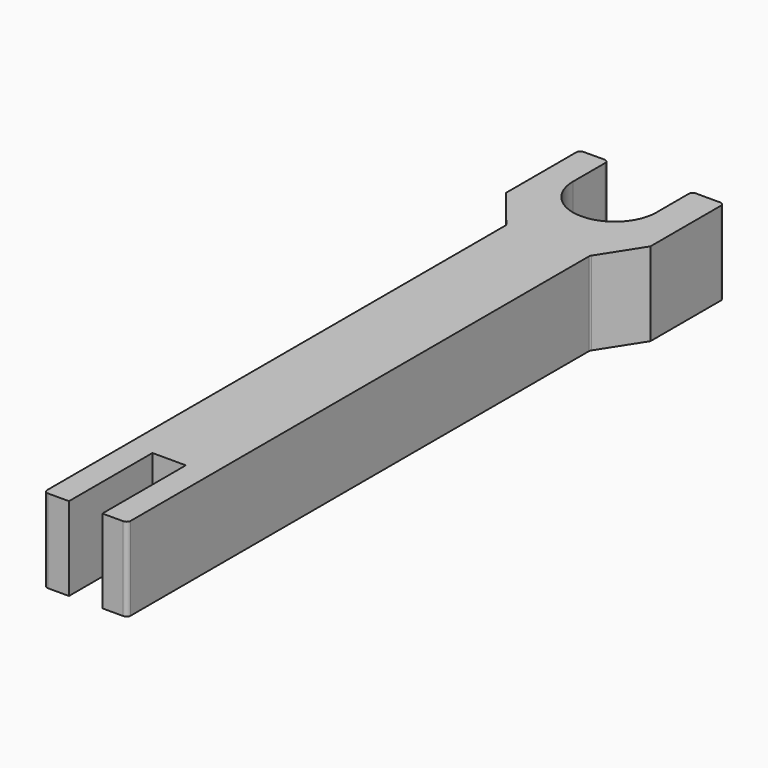
from build123d import *

# Parameters (mm, degrees)
F1_DEPTH = 20
F2_R     = 1
F3_R     = 9.99999


# Not quite as in the source:
# - two fillets or chamfers of one size are made in one step
# - a fillet or chamfer is up to 0.001 mm smaller than in the source, because OpenCascade refuses the exact size


with BuildPart() as f1:
    # F0 (on Top) → F1 (new body)
    with BuildSketch(Plane.XY):
        Polygon((-26.4541809829, 58.4762617946), (-26.4541809829, -79.9982637167), (-20.4541809829, -79.9982637167), (-20.4541809829, -54.9982637167), (-12.4541809829, -54.9982637167), (-12.4541809829, -79.9982637167), (-6.4541809829, -79.9982637167), (-6.4541809829, 58.4762617946), (0, 68.5610547662), (0, 90.617305144), (-7.710005641, 90.617305144), (-7.710005641, 70.0017362833), (-27.710005641, 70.0017362833), (-27.710005641, 90.6515493989), (-34.6441827714, 90.6196484681), (-34.6441827714, 68.5610547662), align=None)
    extrude(amount=F1_DEPTH)

    # F2
    f2_edges = [f1.edges().sort_by_distance(p)[0] for p in [
        (-26.454181, -79.998264, 10),
        (-6.454181, -79.998264, 10),
        (-27.710006, 90.651549, 10),
        (-34.644183, 90.619648, 10),
        (-26.454181, 58.476262, 10),
        (-6.454181, 58.476262, 10),
        (0, 90.617305, 10),
        (-7.710006, 90.617305, 10),
    ]]
    fillet(f2_edges, radius=F2_R)

    # F3 (radius 10 in the source; OpenCascade refuses exactly that, so slightly less here)
    f3_edges = [f1.edges().sort_by_distance(p)[0] for p in [
        (-7.710006, 70.001736, 10),
        (-27.710006, 70.001736, 10),
    ]]
    fillet(f3_edges, radius=F3_R)


solid = f1.part
